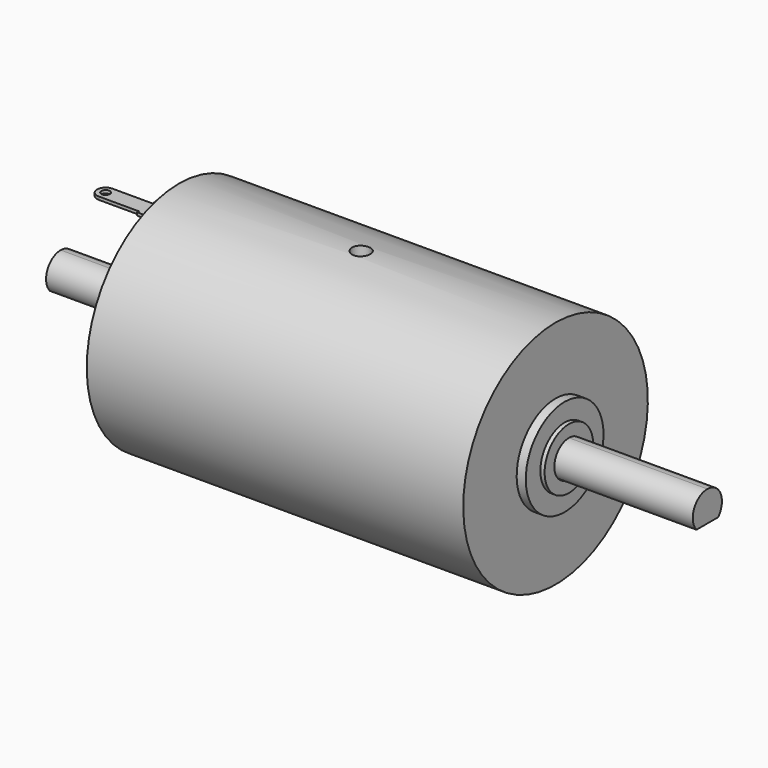
from build123d import *
from build123d import SkipClean  # not in build123d's __all__

# Parameters (mm, degrees)
F5_DEPTH         = 1.27
F5_COPIES2_COUNT = 2
F7_R             = 3.81
F8_DEPTH         = 25.4
F9_R             = 2.54
F10_DEPTH        = 25.4
F9_R_2           = 40.64
F9_W             = 8.89
F9_H             = 1.27
F9_R_3           = 19.05
F11_DEPTH        = 2.54
F12_R            = 48.26
F12_R_2          = 40.64
F13_DEPTH        = 5.08
F15_DEPTH        = 270.51


# Not quite as in the source:
# - after a boolean that leaves OpenCascade's solid faulty, fix() repairs it
# - a pattern or mirror of a feature is missing from the dataset's text; its kind, count and spacing are read off the source's solid


with BuildPart() as f1:
    # F0 (on Front) → F1 (revolve)
    with BuildSketch(Plane.XZ):
        Polygon((-270.51, 0), (0, 0), (0, 7.62), (-57.912, 7.62), (-57.912, 12.7), (-59.69, 12.7), (-59.69, 20.32), (-63.5, 20.32), (-63.5, 48.26), (-226.06, 48.26), (-226.06, 19.05), (-229.87, 19.05), (-229.87, 7.62), (-270.51, 7.62), align=None)
    revolve(axis=Axis((-130.6665660813, 0, 0), (1, 0, 0)))

    # F4 (on offset) → F5 (join)
    with BuildSketch(Plane.XY.offset(34.925)):
        with BuildLine():
            Line((-226.06, 0), (-226.06, 4.445))
            Line((-226.06, 4.445), (-234.95, 4.445))
            Line((-234.95, 4.445), (-234.95, 3.556))
            Line((-234.95, 3.556), (-251.714, 3.556))
            ThreePointArc((-251.714, 3.556), (-254.2284717139, 2.5144717139), (-255.27, 0))
            Line((-255.27, 0), (-253.492, 0))
            ThreePointArc((-253.492, 0), (-251.714, 1.778), (-249.936, 0))
            Line((-249.936, 0), (-226.06, 0))
        make_face()
    f5 = extrude(amount=-F5_DEPTH)

    # F5_copies: F5 across plane
    add(f5.mirror(Plane(origin=(0, 0, 0), x_dir=(-1, 0, 0), z_dir=(0, 0, -1))), clean=False)

    # F5_copies1: F5 across plane
    with SkipClean():  # cleaning this boolean's faces spoils the solid; the shape is the same uncleaned
        add(f5.mirror(Plane(origin=(0, 0, 0), x_dir=(0, 0, -1), z_dir=(0, -1, 0))), clean=False)

    # F5_copies2: F5 ×2 about axis
    f5_copies2_axis = Axis((0, 0, 0), (1, 0, 0))
    with SkipClean():  # cleaning this boolean's faces spoils the solid; the shape is the same uncleaned
        for i in range(1, F5_COPIES2_COUNT):
            add(f5.rotate(f5_copies2_axis, i * 360 / F5_COPIES2_COUNT), clean=False)

    # F7 (on offset) → F8 (cut)
    with BuildSketch(Plane.XY.offset(48.26)):
        with Locations((-144.78, 0)):
            Circle(F7_R)
    extrude(amount=-F8_DEPTH, mode=Mode.SUBTRACT)

    # F9 (on face) → F10 (cut)
    with BuildSketch(Plane(origin=(-226.06, 0, 0), x_dir=(0, -1, 0), z_dir=(-1, 0, 0))):
        with Locations((30.7958633586, 17.78)):
            Circle(F9_R)
        with Locations((-30.7958633586, -17.78)):
            Circle(F9_R)
    extrude(amount=-F10_DEPTH, mode=Mode.SUBTRACT)

    # F9 (on face) → F11 (cut)
    with BuildSketch(Plane(origin=(-226.06, 0, 0), x_dir=(0, -1, 0), z_dir=(-1, 0, 0))):
        Circle(F9_R_2)
        with Locations((-30.7958633586, -17.78)):
            Circle(F9_R, mode=Mode.SUBTRACT)
        with Locations((0, -34.29)):
            Rectangle(F9_W, F9_H, mode=Mode.SUBTRACT)
        Circle(F9_R_3, mode=Mode.SUBTRACT)
        with Locations((30.7958633586, 17.78)):
            Circle(F9_R, mode=Mode.SUBTRACT)
        with Locations((0, 34.29)):
            Rectangle(F9_W, F9_H, mode=Mode.SUBTRACT)
    with SkipClean():  # cleaning this boolean's faces spoils the solid; the shape is the same uncleaned
        extrude(amount=-F11_DEPTH, mode=Mode.SUBTRACT)

    # F12 (on face) → F13 (cut)
    with BuildSketch(Plane(origin=(-226.06, 0, 0), x_dir=(0, -1, 0), z_dir=(-1, 0, 0))):
        Circle(F12_R)
        Circle(F12_R_2, mode=Mode.SUBTRACT)
    extrude(amount=-F13_DEPTH, mode=Mode.SUBTRACT)

    add(f1.part.fix(), mode=Mode.REPLACE)

    # F14 (on face) → F15 (cut, through all)
    with BuildSketch(Plane.YZ):
        with BuildLine():
            Line((5.6796126628, -5.08), (-5.6796126628, -5.08))
            ThreePointArc((-5.6796126628, -5.08), (0, -7.62), (5.6796126628, -5.08))
        make_face()
    extrude(amount=-F15_DEPTH, mode=Mode.SUBTRACT)

    add(f1.part.fix(), mode=Mode.REPLACE)


solid = f1.part
